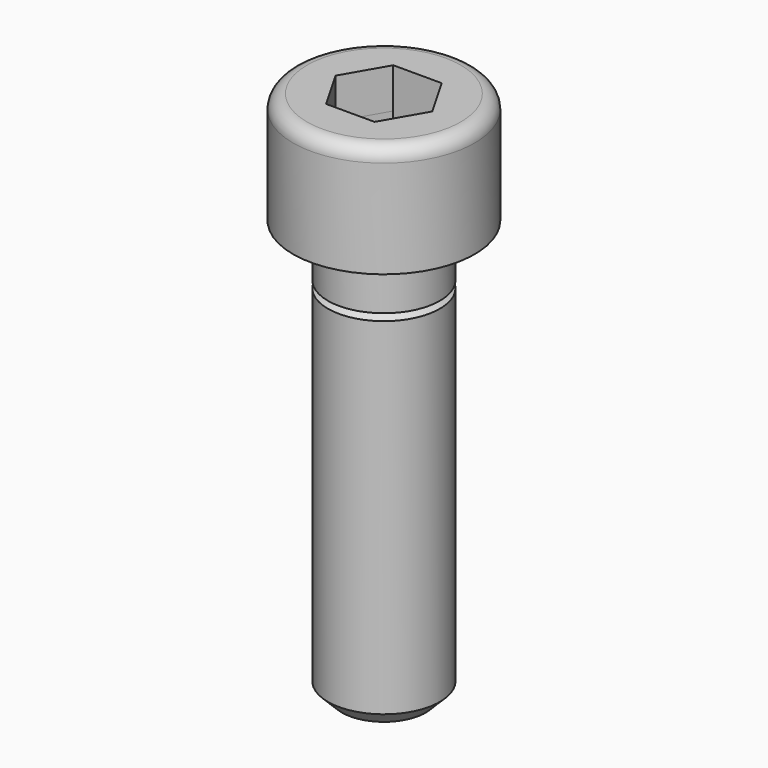
from build123d import *

# Parameters (mm, degrees)
F2_R     = 1
F3_SIZE  = 1
F5_DEPTH = 2.88


# Not quite as in the source:
# - a fillet or chamfer that OpenCascade refuses, or shapes differently, is made with other operations: its cross-section is extruded or revolved along the edge and cut away or added


with BuildPart() as f1:
    # F0 (on Front) → F1 (revolve)
    with BuildSketch(Plane.XZ):
        Polygon((-4, 0), (0, 0), (0, 31.056624327), (-2.5, 32.5), (-2.5, 38), (-6.5, 38), (-6.5, 30), (-4, 30), (-4, 26.25), (-3.5, 26), (-4, 25.75), align=None)
    revolve(axis=Axis((0, 0, 18.332445994), (0, 0, 1)))

    # F2
    f2_edges = [f1.edges().sort_by_distance(p)[0] for p in [
        (6.5, 0, 38),
    ]]
    fillet(f2_edges, radius=F2_R)

    # F3
    f3_edges = [f1.edges().sort_by_distance(p)[0] for p in [
        (4, 0, 0),
    ]]
    chamfer(f3_edges, length=F3_SIZE)

    # F4 (on face) → F5 (cut)
    with BuildSketch(Plane.XY.offset(38)):
        Polygon((-1.7320508076, -3), (1.7320508076, -3), (3.4641016151, 0), (1.7320508076, 3), (-1.7320508076, 3), (-3.4641016151, 0), align=None)
    extrude(amount=-F5_DEPTH, mode=Mode.SUBTRACT)

    # F6: chamfer of 1.5 x 2.5980762114 on 1 edges, made by hand


with BuildPart() as f6_tool2:
    # F6_s3 → F6_t4 (revolve)
    with BuildSketch(Plane.XZ):
        Polygon((-5.0980762114, 35.12), (-2.5, 33.62), (-2.5, 35.12), align=None)
    revolve(axis=Axis((0, 0, 35.12), (0, 0, 1)))

    split(bisect_by=Plane(origin=(-2.5980762114, -1.5, 0), x_dir=(0, 0, 1), z_dir=(0.8660254038, 0.5, 0)), keep=Keep.TOP)

    split(bisect_by=Plane(origin=(-2.5980762114, 1.5, 0), x_dir=(0, 0, 1), z_dir=(0.8660254038, -0.5, 0)), keep=Keep.TOP)

    split(bisect_by=Plane.XZ.offset(-3), keep=Keep.TOP)

    split(bisect_by=Plane(origin=(2.5980762114, 1.5, 0), x_dir=(0, 0, 1), z_dir=(-0.8660254038, -0.5, 0)), keep=Keep.TOP)

    split(bisect_by=Plane(origin=(2.5980762114, -1.5, 0), x_dir=(0, 0, 1), z_dir=(-0.8660254038, 0.5, 0)), keep=Keep.TOP)

    split(bisect_by=Plane.XZ.offset(3), keep=Keep.BOTTOM)


with BuildPart() as f1_1:
    add(f1.part)

    # F6_t1: cut F6_tool2
    add(f6_tool2.part, mode=Mode.SUBTRACT)


solid = f1_1.part
